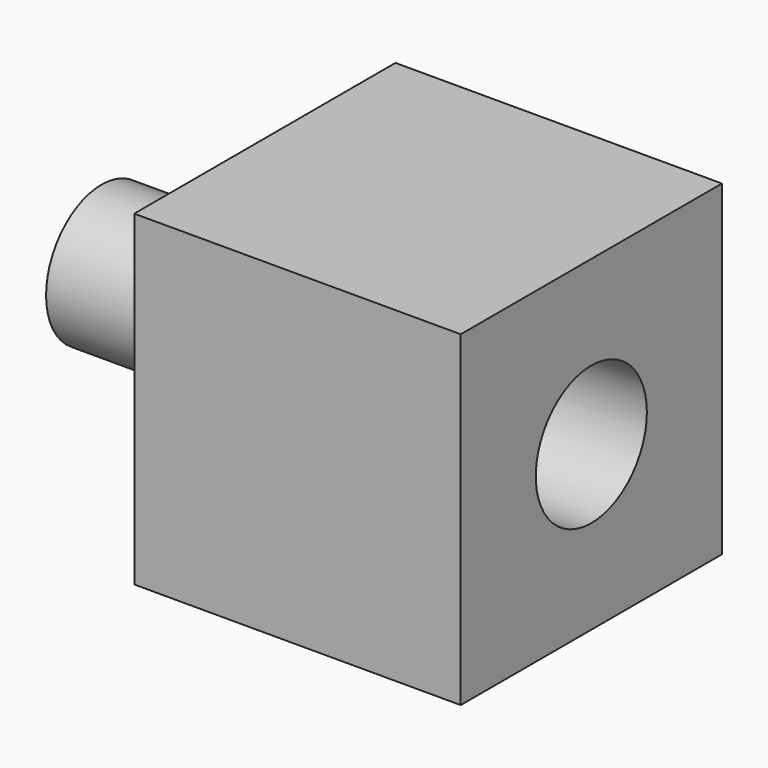
from build123d import *

# Parameters (mm, degrees)
F1_W     = 101.6
F1_H     = 101.6
F2_DEPTH = 50.8
F3_R     = 21.6021439773
F4_DEPTH = 50.8
F5_R     = 21.6021439773
F6_DEPTH = 50.8


# Not quite as in the source:
# - a variable given as a bare number and used for a length is read in inches; the dataset says mm whatever the document's units were


with BuildPart() as f2:
    # F1 (on Front) → F2 (new body, symmetric)
    with BuildSketch(Plane.XZ):
        Rectangle(F1_W, F1_H)
    extrude(amount=F2_DEPTH, both=True)

    # F3 (on face) → F4 (cut)
    with BuildSketch(Plane.YZ.offset(50.8)):
        Circle(F3_R)
    extrude(amount=-F4_DEPTH, mode=Mode.SUBTRACT)

    # F5 (on face) → F6 (join)
    with BuildSketch(Plane(origin=(-50.8, 0, 0), x_dir=(0, -1, 0), z_dir=(-1, 0, 0))):
        Circle(F5_R)
    extrude(amount=F6_DEPTH)


solid = f2.part
